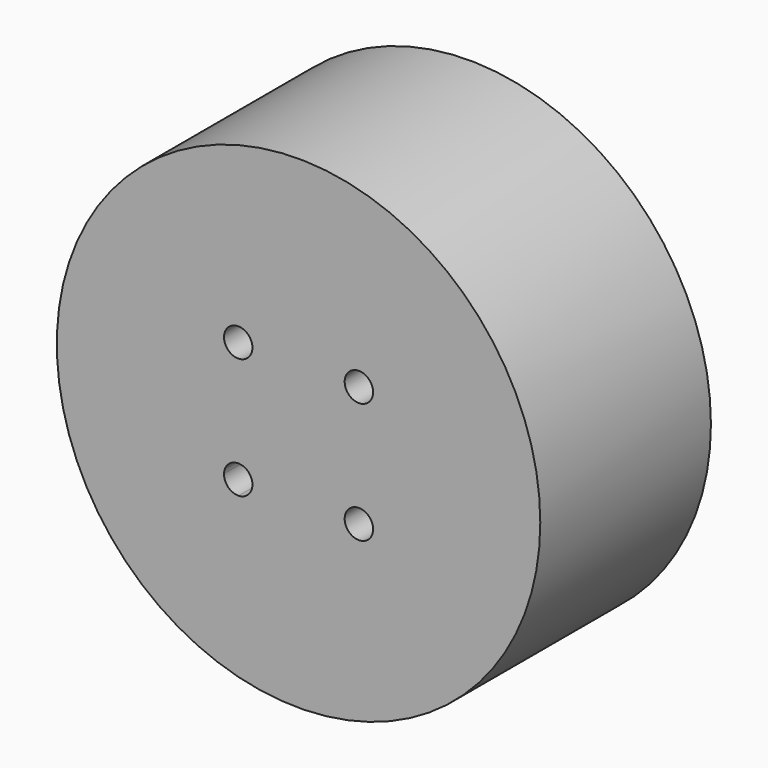
from build123d import *

# Parameters (mm, degrees)
F0_R     = 17
F0_R_2   = 1.5
F0_R_3   = 1
F0_R_4   = 4
F0_R_5   = 1.475
F1_DEPTH = 15
F2_START = 10
F2_DEPTH = 15
F3_DEPTH = 5
F4_DEPTH = 0.6
F5_DEPTH = 1.2


# Not quite as in the source:
# - a feature names something its author has since deleted; it is built from what else it names


with BuildPart() as f1:
    # F0 (on Front) → F1 (new body)
    with BuildSketch(Plane.XZ):
        Circle(F0_R)
        with BuildLine():
            ThreePointArc((-4.2152867015, -5.2422664968), (-4.1715341961, -5.447511614), (-4.1568542495, -5.6568542495))
            ThreePointArc((-4.1568542495, -5.6568542495), (-6.8551617286, -6.5591065343), (-5.2422664968, -4.2152867015))
            ThreePointArc((-5.2422664968, -4.2152867015), (-4.2289624147, -3.2427342391), (-3.2426406871, -4.2426406871))
            ThreePointArc((-3.2426406871, -4.2426406871), (-3.525928058, -4.9400093179), (-4.2152867015, -5.2422664968))
        make_face(mode=Mode.SUBTRACT)
        with Locations((6.7175144213, -6.7175144213)):
            Circle(F0_R_2, mode=Mode.SUBTRACT)
        with Locations((4.2426406871, -4.2426406871)):
            Circle(F0_R_3, mode=Mode.SUBTRACT)
        with Locations((-4.2426406871, 4.2426406871)):
            Circle(F0_R_3, mode=Mode.SUBTRACT)
        with Locations((-6.7175144213, 6.7175144213)):
            Circle(F0_R_2, mode=Mode.SUBTRACT)
        Circle(F0_R_4, mode=Mode.SUBTRACT)
        with BuildLine():
            ThreePointArc((4.2152867015, 5.2422664968), (5.447511614, 7.1421743029), (7.1568542495, 5.6568542495))
            ThreePointArc((7.1568542495, 5.6568542495), (6.5591065343, 4.4585467704), (5.2422664968, 4.2152867015))
            ThreePointArc((5.2422664968, 4.2152867015), (3.5355339059, 3.5355339059), (4.2152867015, 5.2422664968))
        make_face(mode=Mode.SUBTRACT)
        with BuildLine():
            ThreePointArc((5.2422664968, 4.2152867015), (6.5591065343, 4.4585467704), (7.1568542495, 5.6568542495))
            ThreePointArc((7.1568542495, 5.6568542495), (5.447511614, 7.1421743029), (4.2152867015, 5.2422664968))
            ThreePointArc((4.2152867015, 5.2422664968), (4.9400093179, 4.9593533163), (5.2426406871, 4.2426406871))
            ThreePointArc((5.2426406871, 4.2426406871), (5.2425471352, 4.2289624147), (5.2422664968, 4.2152867015))
        make_face()
        with BuildLine():
            ThreePointArc((5.2422664968, 4.2152867015), (4.5961940777, 4.5961940777), (4.2152867015, 5.2422664968))
            ThreePointArc((4.2152867015, 5.2422664968), (3.5355339059, 3.5355339059), (5.2422664968, 4.2152867015))
        make_face()
        with BuildLine():
            ThreePointArc((-5.2422664968, -4.2152867015), (-6.8551617286, -6.5591065343), (-4.1568542495, -5.6568542495))
            ThreePointArc((-4.1568542495, -5.6568542495), (-4.1715341961, -5.447511614), (-4.2152867015, -5.2422664968))
            ThreePointArc((-4.2152867015, -5.2422664968), (-4.9497474683, -4.9497474683), (-5.2422664968, -4.2152867015))
        make_face()
        with BuildLine():
            ThreePointArc((-5.2422664968, -4.2152867015), (-4.9497474683, -4.9497474683), (-4.2152867015, -5.2422664968))
            ThreePointArc((-4.2152867015, -5.2422664968), (-4.5961940777, -4.5961940777), (-5.2422664968, -4.2152867015))
        make_face()
        with BuildLine():
            ThreePointArc((-5.2422664968, -4.2152867015), (-4.5961940777, -4.5961940777), (-4.2152867015, -5.2422664968))
            ThreePointArc((-4.2152867015, -5.2422664968), (-3.525928058, -4.9400093179), (-3.2426406871, -4.2426406871))
            ThreePointArc((-3.2426406871, -4.2426406871), (-4.2289624147, -3.2427342391), (-5.2422664968, -4.2152867015))
        make_face()
        with BuildLine():
            ThreePointArc((5.2426406871, 4.2426406871), (4.9400093179, 4.9593533163), (4.2152867015, 5.2422664968))
            ThreePointArc((4.2152867015, 5.2422664968), (4.5961940777, 4.5961940777), (5.2422664968, 4.2152867015))
            ThreePointArc((5.2422664968, 4.2152867015), (5.2425471352, 4.2289624147), (5.2426406871, 4.2426406871))
        make_face()
        with Locations((4.2426406871, -4.2426406871)):
            Circle(F0_R_3)
        with Locations((-4.2426406871, 4.2426406871)):
            Circle(F0_R_3)
        with Locations((-6.7175144213, 6.7175144213)):
            Circle(F0_R_2)
        with Locations((6.7175144213, -6.7175144213)):
            Circle(F0_R_2)
        Circle(F0_R_4)
        Circle(F0_R_5, mode=Mode.SUBTRACT)
        Circle(F0_R_5)
    extrude(amount=F1_DEPTH)

    # F0 (on Front) → F2 (cut)
    with BuildSketch(Plane.XZ.offset(F2_START)):
        with BuildLine():
            ThreePointArc((-5.2422664968, -4.2152867015), (-4.5961940777, -4.5961940777), (-4.2152867015, -5.2422664968))
            ThreePointArc((-4.2152867015, -5.2422664968), (-3.525928058, -4.9400093179), (-3.2426406871, -4.2426406871))
            ThreePointArc((-3.2426406871, -4.2426406871), (-4.2289624147, -3.2427342391), (-5.2422664968, -4.2152867015))
        make_face()
        with BuildLine():
            ThreePointArc((-5.2422664968, -4.2152867015), (-4.9497474683, -4.9497474683), (-4.2152867015, -5.2422664968))
            ThreePointArc((-4.2152867015, -5.2422664968), (-4.5961940777, -4.5961940777), (-5.2422664968, -4.2152867015))
        make_face()
        with Locations((4.2426406871, -4.2426406871)):
            Circle(F0_R_3)
        with BuildLine():
            ThreePointArc((5.2422664968, 4.2152867015), (4.5961940777, 4.5961940777), (4.2152867015, 5.2422664968))
            ThreePointArc((4.2152867015, 5.2422664968), (3.5355339059, 3.5355339059), (5.2422664968, 4.2152867015))
        make_face()
        with BuildLine():
            ThreePointArc((5.2426406871, 4.2426406871), (4.9400093179, 4.9593533163), (4.2152867015, 5.2422664968))
            ThreePointArc((4.2152867015, 5.2422664968), (4.5961940777, 4.5961940777), (5.2422664968, 4.2152867015))
            ThreePointArc((5.2422664968, 4.2152867015), (5.2425471352, 4.2289624147), (5.2426406871, 4.2426406871))
        make_face()
        with Locations((-4.2426406871, 4.2426406871)):
            Circle(F0_R_3)
    extrude(amount=F2_DEPTH, mode=Mode.SUBTRACT)

    # F0 (on Front) → F3 (cut)
    with BuildSketch(Plane.XZ):
        with BuildLine():
            ThreePointArc((5.2422664968, 4.2152867015), (6.5591065343, 4.4585467704), (7.1568542495, 5.6568542495))
            ThreePointArc((7.1568542495, 5.6568542495), (5.447511614, 7.1421743029), (4.2152867015, 5.2422664968))
            ThreePointArc((4.2152867015, 5.2422664968), (4.9400093179, 4.9593533163), (5.2426406871, 4.2426406871))
            ThreePointArc((5.2426406871, 4.2426406871), (5.2425471352, 4.2289624147), (5.2422664968, 4.2152867015))
        make_face()
        with BuildLine():
            ThreePointArc((5.2426406871, 4.2426406871), (4.9400093179, 4.9593533163), (4.2152867015, 5.2422664968))
            ThreePointArc((4.2152867015, 5.2422664968), (4.5961940777, 4.5961940777), (5.2422664968, 4.2152867015))
            ThreePointArc((5.2422664968, 4.2152867015), (5.2425471352, 4.2289624147), (5.2426406871, 4.2426406871))
        make_face()
        with BuildLine():
            ThreePointArc((-5.2422664968, -4.2152867015), (-6.8551617286, -6.5591065343), (-4.1568542495, -5.6568542495))
            ThreePointArc((-4.1568542495, -5.6568542495), (-4.1715341961, -5.447511614), (-4.2152867015, -5.2422664968))
            ThreePointArc((-4.2152867015, -5.2422664968), (-4.9497474683, -4.9497474683), (-5.2422664968, -4.2152867015))
        make_face()
        with BuildLine():
            ThreePointArc((-5.2422664968, -4.2152867015), (-4.9497474683, -4.9497474683), (-4.2152867015, -5.2422664968))
            ThreePointArc((-4.2152867015, -5.2422664968), (-4.5961940777, -4.5961940777), (-5.2422664968, -4.2152867015))
        make_face()
        with Locations((6.7175144213, -6.7175144213)):
            Circle(F0_R_2)
        with Locations((-6.7175144213, 6.7175144213)):
            Circle(F0_R_2)
    extrude(amount=F3_DEPTH, mode=Mode.SUBTRACT)

    # F0 (on Front) → F4 (join)
    with BuildSketch(Plane.XZ):
        Circle(F0_R_4)
        Circle(F0_R_5, mode=Mode.SUBTRACT)
    extrude(amount=-F4_DEPTH)

    # F0 (on Front) → F5 (join)
    with BuildSketch(Plane.XZ):
        Circle(F0_R_5)
    extrude(amount=-F5_DEPTH)


solid = f1.part
